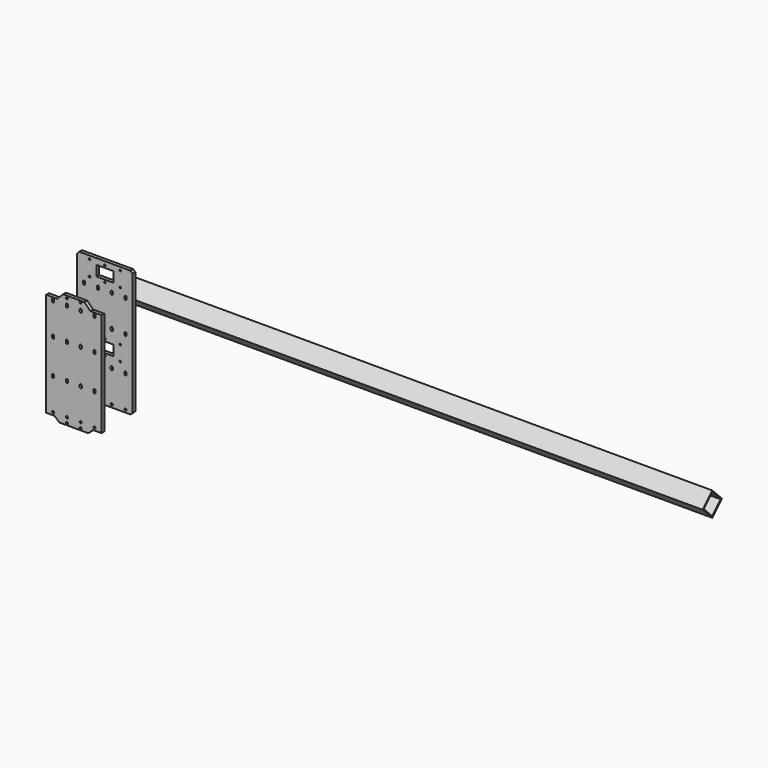
from build123d import *

# Parameters (mm, degrees)
F2_DEPTH = 1380
F3_T     = -2.5
F4_R     = 2.5
F4_R_2   = 2.5703929726
F4_R_3   = 2.4889347238
F5_DEPTH = 8
F7_R     = 2.5
F7_R_2   = 2.05
F7_W     = 40
F7_H     = 24
F8_DEPTH = 8


# Not quite as in the source:
# - a feature names something its author has since deleted; it is built from what else it names


with BuildPart() as f2:
    # F1 (on Right) → F2 (new body)
    with BuildSketch(Plane.YZ):
        Polygon((165.6129737569, 100.5009111076), (137.3287025094, 128.785182355), (109.0444312619, 100.5009111076), (137.3287025094, 72.2166398601), align=None)
    extrude(amount=F2_DEPTH)

    # F3
    f3_openings = [f2.faces().sort_by_distance(p)[0] for p in [
        (0, 137.328703, 100.500911),
        (1380, 137.328703, 100.500911),
    ]]
    offset(amount=F3_T, openings=f3_openings)


with BuildPart() as f5:
    # F4 (on Front) → F5 (new body)
    with BuildSketch(Plane.XZ):
        Polygon((65, -121.7), (65, 121.7), (39, 121.7), (-39, 121.7), (-65, 121.7), (-65, -121.7), (-45, -121.7), (-34, -131.8), (34, -131.8), (45, -121.7), align=None)
        with Locations((-48.5, -115.09)):
            Circle(F4_R, mode=Mode.SUBTRACT)
        with Locations((-16.18, -127.59)):
            Circle(F4_R, mode=Mode.SUBTRACT)
        with Locations((-16.18, -115.09)):
            Circle(F4_R, mode=Mode.SUBTRACT)
        with BuildLine():
            Line((-46, -38.512), (-46, -42.512))
            ThreePointArc((-46, -42.512), (-48.5, -45.012), (-51, -42.512))
            Line((-51, -42.512), (-51, -38.512))
            ThreePointArc((-51, -38.512), (-48.5, -36.012), (-46, -38.512))
        make_face(mode=Mode.SUBTRACT)
        with BuildLine():
            Line((-13.68, -38.512), (-13.68, -42.512))
            ThreePointArc((-13.68, -42.512), (-16.18, -45.012), (-18.68, -42.512))
            Line((-18.68, -42.512), (-18.68, -38.512))
            ThreePointArc((-18.68, -38.512), (-16.18, -36.012), (-13.68, -38.512))
        make_face(mode=Mode.SUBTRACT)
        with Locations((16.18, -127.59)):
            Circle(F4_R, mode=Mode.SUBTRACT)
        with Locations((16.18, -115.09)):
            Circle(F4_R, mode=Mode.SUBTRACT)
        with Locations((48.5, -115.09)):
            Circle(F4_R, mode=Mode.SUBTRACT)
        with BuildLine():
            Line((18.68, -38.512), (18.68, -42.512))
            ThreePointArc((18.68, -42.512), (16.18, -45.012), (13.68, -42.512))
            Line((13.68, -42.512), (13.68, -38.512))
            ThreePointArc((13.68, -38.512), (16.18, -36.012), (18.68, -38.512))
        make_face(mode=Mode.SUBTRACT)
        with BuildLine():
            Line((51, -38.512), (51, -42.512))
            ThreePointArc((51, -42.512), (48.5, -45.012), (46, -42.512))
            Line((46, -42.512), (46, -38.512))
            ThreePointArc((46, -38.512), (48.5, -36.012), (51, -38.512))
        make_face(mode=Mode.SUBTRACT)
        with BuildLine():
            Line((-51, 38.512), (-51, 42.512))
            ThreePointArc((-51, 42.512), (-48.5, 45.012), (-46, 42.512))
            Line((-46, 42.512), (-46, 38.512))
            ThreePointArc((-46, 38.512), (-48.5, 36.012), (-51, 38.512))
        make_face(mode=Mode.SUBTRACT)
        with BuildLine():
            Line((-18.68, 38.512), (-18.68, 42.512))
            ThreePointArc((-18.68, 42.512), (-16.18, 45.012), (-13.68, 42.512))
            Line((-13.68, 42.512), (-13.68, 38.512))
            ThreePointArc((-13.68, 38.512), (-16.18, 36.012), (-18.68, 38.512))
        make_face(mode=Mode.SUBTRACT)
        with BuildLine():
            Line((-51, 113.09), (-51, 117.09))
            ThreePointArc((-51, 117.09), (-48.5, 119.59), (-46, 117.09))
            Line((-46, 117.09), (-46, 113.09))
            ThreePointArc((-46, 113.09), (-48.5, 110.59), (-51, 113.09))
        make_face(mode=Mode.SUBTRACT)
        with BuildLine():
            Line((-18.68, 113.09), (-18.68, 117.09))
            ThreePointArc((-18.68, 117.09), (-16.18, 119.59), (-13.68, 117.09))
            Line((-13.68, 117.09), (-13.68, 113.09))
            ThreePointArc((-13.68, 113.09), (-16.18, 110.59), (-18.68, 113.09))
        make_face(mode=Mode.SUBTRACT)
        with BuildLine():
            Line((13.68, 38.512), (13.68, 42.512))
            ThreePointArc((13.68, 42.512), (16.18, 45.012), (18.68, 42.512))
            Line((18.68, 42.512), (18.68, 38.512))
            ThreePointArc((18.68, 38.512), (16.18, 36.012), (13.68, 38.512))
        make_face(mode=Mode.SUBTRACT)
        with BuildLine():
            Line((46, 38.512), (46, 42.512))
            ThreePointArc((46, 42.512), (48.5, 45.012), (51, 42.512))
            Line((51, 42.512), (51, 38.512))
            ThreePointArc((51, 38.512), (48.5, 36.012), (46, 38.512))
        make_face(mode=Mode.SUBTRACT)
        with BuildLine():
            Line((13.68, 113.09), (13.68, 117.09))
            ThreePointArc((13.68, 117.09), (16.18, 119.59), (18.68, 117.09))
            Line((18.68, 117.09), (18.68, 113.09))
            ThreePointArc((18.68, 113.09), (16.18, 110.59), (13.68, 113.09))
        make_face(mode=Mode.SUBTRACT)
        with BuildLine():
            Line((46, 113.09), (46, 117.09))
            ThreePointArc((46, 117.09), (48.5, 119.59), (51, 117.09))
            Line((51, 117.09), (51, 113.09))
            ThreePointArc((51, 113.09), (48.5, 110.59), (46, 113.09))
        make_face(mode=Mode.SUBTRACT)
        Polygon((-39, 121.7), (39, 121.7), (25, 135.7), (-25, 135.7), align=None)
        with Locations((-16.18, 130.7444572449)):
            Circle(F4_R_2, mode=Mode.SUBTRACT)
        with Locations((16.18, 132.09)):
            Circle(F4_R_3, mode=Mode.SUBTRACT)
    extrude(amount=F5_DEPTH)


with BuildPart() as f8:
    # F7 (on offset) → F8 (new body)
    with BuildSketch(Plane.XZ.offset(-83)):
        Polygon((60, 175.09), (-60, 175.09), (-65, 170.09), (-65, -116.7), (-60, -121.7), (60, -121.7), (65, -116.7), (65, 170.09), align=None)
        with Locations((-48.51, -115.2)):
            Circle(F7_R, mode=Mode.SUBTRACT)
        with Locations((-16.17, -115.2)):
            Circle(F7_R, mode=Mode.SUBTRACT)
        with BuildLine():
            Line((-46.01, -38.73), (-46.01, -42.73))
            ThreePointArc((-46.01, -42.73), (-48.51, -45.23), (-51.01, -42.73))
            Line((-51.01, -42.73), (-51.01, -38.9570118877))
            ThreePointArc((-51.01, -38.9570118877), (-48.6287763125, -36.2274246067), (-46.01, -38.73))
        make_face(mode=Mode.SUBTRACT)
        with Locations((-36, -20)):
            Circle(F7_R_2, mode=Mode.SUBTRACT)
        with Locations((-36, 15)):
            Circle(F7_R_2, mode=Mode.SUBTRACT)
        with BuildLine():
            Line((-13.67, -38.73), (-13.67, -42.73))
            ThreePointArc((-13.67, -42.73), (-16.17, -45.23), (-18.67, -42.73))
            Line((-18.67, -42.73), (-18.67, -39.0080270306))
            ThreePointArc((-18.67, -39.0080270306), (-16.3169581646, -36.2261380315), (-13.67, -38.73))
        make_face(mode=Mode.SUBTRACT)
        with Locations((16.17, -115.2)):
            Circle(F7_R, mode=Mode.SUBTRACT)
        with Locations((48.51, -115.2)):
            Circle(F7_R, mode=Mode.SUBTRACT)
        with BuildLine():
            Line((18.67, -38.73), (18.67, -42.73))
            ThreePointArc((18.67, -42.73), (16.17, -45.23), (13.67, -42.73))
            Line((13.67, -42.73), (13.67, -39.0075720796))
            ThreePointArc((13.67, -39.0075720796), (13.6584102142, -38.8690010606), (13.6545429641, -38.73))
            ThreePointArc((13.6545429641, -38.73), (16.1545429641, -36.23), (18.6545429641, -38.73))
            Line((18.6545429641, -38.73), (18.67, -38.73))
        make_face(mode=Mode.SUBTRACT)
        with Locations((0, -20)):
            Circle(F7_R_2, mode=Mode.SUBTRACT)
        with Locations((0, -2.5)):
            Rectangle(F7_W, F7_H, mode=Mode.SUBTRACT)
        with Locations((0, 15)):
            Circle(F7_R_2, mode=Mode.SUBTRACT)
        with BuildLine():
            Line((51.01, -42.7297875421), (51.01, -42.73))
            ThreePointArc((51.01, -42.73), (48.1449929341, -45.2503029403), (46.01, -42.0877094524))
            Line((46.01, -42.0877094524), (46.01, -38.73))
            ThreePointArc((46.01, -38.73), (48.51, -36.23), (51.01, -38.73))
            Line((51.01, -38.73), (51.01, -42.7297875421))
        make_face(mode=Mode.SUBTRACT)
        with Locations((36, -20)):
            Circle(F7_R_2, mode=Mode.SUBTRACT)
        with Locations((36, 15)):
            Circle(F7_R_2, mode=Mode.SUBTRACT)
        with BuildLine():
            Line((-46.01, 42.0886284048), (-46.01, 38.512))
            ThreePointArc((-46.01, 38.512), (-48.51, 36.012), (-51.01, 38.512))
            ThreePointArc((-51.01, 38.512), (-51.0009654295, 38.7243469541), (-50.9739270169, 38.9351591373))
            Line((-50.9739270169, 38.9351591373), (-50.9739270169, 42.5117875421))
            ThreePointArc((-50.9739270169, 42.5117875421), (-48.4739270169, 45.0117875421), (-45.9739270169, 42.5117875421))
            ThreePointArc((-45.9739270169, 42.5117875421), (-45.9829615873, 42.299440588), (-46.01, 42.0886284048))
        make_face(mode=Mode.SUBTRACT)
        with BuildLine():
            Line((-13.67, 42.1039142989), (-13.67, 38.512))
            ThreePointArc((-13.67, 38.512), (-16.17, 36.012), (-18.67, 38.512))
            ThreePointArc((-18.67, 38.512), (-18.6616117976, 38.7166231899), (-18.6365034801, 38.9198732432))
            Line((-18.6365034801, 38.9198732432), (-18.6365034801, 42.5117875421))
            ThreePointArc((-18.6365034801, 42.5117875421), (-16.1365034801, 45.0117875421), (-13.6365034801, 42.5117875421))
            ThreePointArc((-13.6365034801, 42.5117875421), (-13.6448916825, 42.3071643522), (-13.67, 42.1039142989))
        make_face(mode=Mode.SUBTRACT)
        with BuildLine():
            Line((-51.01, 113.09), (-51.01, 116.9834371618))
            ThreePointArc((-51.01, 116.9834371618), (-48.5632935076, 119.5917025084), (-46.007729903, 117.09))
            Line((-46.007729903, 117.09), (-46.007729903, 113.09))
            ThreePointArc((-46.007729903, 113.09), (-48.507729903, 110.59), (-51.007729903, 113.09))
            Line((-51.007729903, 113.09), (-51.01, 113.09))
        make_face(mode=Mode.SUBTRACT)
        with Locations((-36, 131.59)):
            Circle(F7_R_2, mode=Mode.SUBTRACT)
        with Locations((-36, 167.59)):
            Circle(F7_R_2, mode=Mode.SUBTRACT)
        with BuildLine():
            ThreePointArc((-13.667729903, 113.09), (-16.167729903, 110.59), (-18.667729903, 113.09))
            Line((-18.667729903, 113.09), (-18.67, 113.09))
            Line((-18.67, 113.09), (-18.67, 116.9834371618))
            ThreePointArc((-18.67, 116.9834371618), (-16.2232935076, 119.5917025084), (-13.667729903, 117.09))
            Line((-13.667729903, 117.09), (-13.667729903, 113.09))
        make_face(mode=Mode.SUBTRACT)
        with BuildLine():
            Line((18.67, 42.1537611834), (18.67, 38.512))
            ThreePointArc((18.67, 38.512), (16.17, 36.012), (13.67, 38.512))
            ThreePointArc((13.67, 38.512), (13.676450669, 38.6914762762), (13.695769387, 38.8700263587))
            Line((13.695769387, 38.8700263587), (13.695769387, 42.5117875421))
            ThreePointArc((13.695769387, 42.5117875421), (16.195769387, 45.0117875421), (18.695769387, 42.5117875421))
            ThreePointArc((18.695769387, 42.5117875421), (18.689318718, 42.3323112659), (18.67, 42.1537611834))
        make_face(mode=Mode.SUBTRACT)
        with BuildLine():
            Line((51.01, 42.0596454226), (51.01, 38.512))
            ThreePointArc((51.01, 38.512), (48.51, 36.012), (46.01, 38.512))
            ThreePointArc((46.01, 38.512), (46.020327939, 38.7390088733), (46.0512264229, 38.9641421196))
            Line((46.0512264229, 38.9641421196), (46.0512264229, 42.5117875421))
            ThreePointArc((46.0512264229, 42.5117875421), (48.5512264228, 45.0117875421), (51.0512264228, 42.5117875421))
            ThreePointArc((51.0512264228, 42.5117875421), (51.0408984839, 42.2847786688), (51.01, 42.0596454226))
        make_face(mode=Mode.SUBTRACT)
        with BuildLine():
            ThreePointArc((18.68, 113.09), (16.18, 110.59), (13.68, 113.09))
            Line((13.68, 113.09), (13.67, 113.09))
            Line((13.67, 113.09), (13.67, 116.8124279204))
            ThreePointArc((13.67, 116.8124279204), (13.6584102142, 116.9509989394), (13.6545429641, 117.09))
            ThreePointArc((13.6545429641, 117.09), (16.1545429641, 119.59), (18.6545429641, 117.09))
            Line((18.6545429641, 117.09), (18.67, 117.09))
            Line((18.67, 117.09), (18.68, 117.09))
            Line((18.68, 117.09), (18.68, 113.09))
        make_face(mode=Mode.SUBTRACT)
        with Locations((0, 131.59)):
            Circle(F7_R_2, mode=Mode.SUBTRACT)
        with Locations((0, 149.09)):
            Rectangle(F7_W, F7_H, mode=Mode.SUBTRACT)
        with Locations((0, 166.59)):
            Circle(F7_R_2, mode=Mode.SUBTRACT)
        with BuildLine():
            Line((51.01, 117.09), (51.01, 113.09))
            ThreePointArc((51.01, 113.09), (48.51, 110.59), (46.01, 113.09))
            Line((46.01, 113.09), (46.01, 117.09))
            ThreePointArc((46.01, 117.09), (48.51, 119.59), (51.01, 117.09))
        make_face(mode=Mode.SUBTRACT)
        with Locations((36, 132.59)):
            Circle(F7_R_2, mode=Mode.SUBTRACT)
        with Locations((36, 167.59)):
            Circle(F7_R_2, mode=Mode.SUBTRACT)
    extrude(amount=-F8_DEPTH)


solid = Compound([f2.part, f5.part, f8.part])
